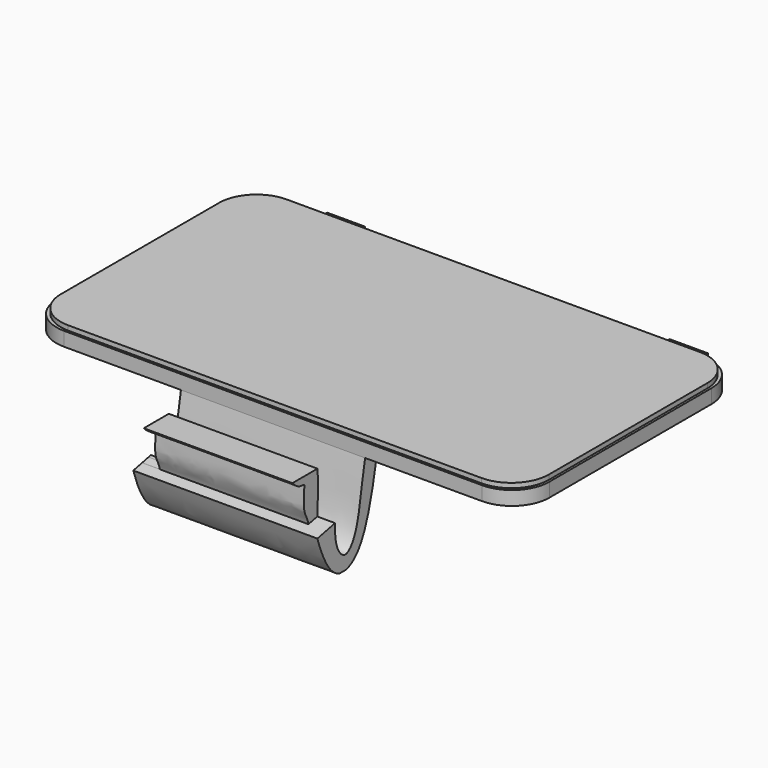
from build123d import *

# Parameters (mm, degrees)
F1_DEPTH  = 1.5
F3_DEPTH  = 0.5
F4_W      = 4.08
F4_H      = 3
F4_H_2    = 2
F5_DEPTH  = 2.15
F4_W_2    = 19.71
F4_H_3    = 8.35
F4_H_4    = 1.65
F6_DEPTH  = 9.5
F8_DEPTH  = 25.4
F9_DEPTH  = 25.4
F10_DEPTH = 25.4
F11_DEPTH = 25.4
F12_DEPTH = 1.9
F14_DEPTH = 1.9
F15_R     = 0.5


with BuildPart() as f1:
    # F0 (on Top) → F1 (new body)
    with BuildSketch(Plane.XY):
        with BuildLine():
            ThreePointArc((26.375, 10.85), (25.2034271247, 13.6784271247), (22.375, 14.85))
            Line((22.375, 14.85), (-22.375, 14.85))
            ThreePointArc((-22.375, 14.85), (-25.2034271247, 13.6784271247), (-26.375, 10.85))
            Line((-26.375, 10.85), (-26.375, -10.85))
            ThreePointArc((-26.375, -10.85), (-25.2034271247, -13.6784271247), (-22.375, -14.85))
            Line((-22.375, -14.85), (22.375, -14.85))
            ThreePointArc((22.375, -14.85), (25.2034271247, -13.6784271247), (26.375, -10.85))
            Line((26.375, -10.85), (26.375, 10.85))
        make_face()
    extrude(amount=F1_DEPTH)

    # F2 (on face) → F3 (join)
    with BuildSketch(Plane.XY.offset(1.5)):
        with BuildLine():
            ThreePointArc((26.125, 10.6), (24.9534271247, 13.4284271247), (22.125, 14.6))
            Line((22.125, 14.6), (-22.125, 14.6))
            ThreePointArc((-22.125, 14.6), (-24.9534271247, 13.4284271247), (-26.125, 10.6))
            Line((-26.125, 10.6), (-26.125, -10.6))
            ThreePointArc((-26.125, -10.6), (-24.9534271247, -13.4284271247), (-22.125, -14.6))
            Line((-22.125, -14.6), (22.125, -14.6))
            ThreePointArc((22.125, -14.6), (24.9534271247, -13.4284271247), (26.125, -10.6))
            Line((26.125, -10.6), (26.125, 10.6))
        make_face()
    extrude(amount=F3_DEPTH)

    # F4 (on face) → F5 (join)
    with BuildSketch(Plane.XY):
        with Locations((-18.335, 16.35)):
            Rectangle(F4_W, F4_H)
        with Locations((-18.335, 13.85)):
            Rectangle(F4_W, F4_H_2)
        with Locations((18.335, 13.85)):
            Rectangle(F4_W, F4_H_2)
        with Locations((18.335, 16.35)):
            Rectangle(F4_W, F4_H)
    extrude(amount=-F5_DEPTH)

    # F4 (on face) → F6 (join)
    with BuildSketch(Plane.XY):
        with Locations((0, -19.025)):
            Rectangle(F4_W_2, F4_H_3)
        with Locations((0, -14.025)):
            Rectangle(F4_W_2, F4_H_4)
    extrude(amount=-F6_DEPTH)

    # F7 (on face) → F8 (cut)
    with BuildSketch(Plane.YZ.offset(9.855)):
        with BuildLine():
            add(Edge.make_bspline(
                [(-18.2, -9.5), (-19.0467439554, -9.3105263347), (-20.1329314913, -7.9995740948), (-20.9745336298, -5.8262032925), (-21.2309185806, -5)],
                knots=[0.5048432027, 0.5048432027, 0.5048432027, 0.5048432027, 0.6991234522, 0.8042040894, 0.8042040894, 0.8042040894, 0.8042040894], degree=3))
            add(Edge.make_bspline(
                [(-21.2309185806, -5), (-21.7086386079, -3.4605420158), (-22.0508473288, -1.7012665692), (-22.2, 0)],
                knots=[0.8042040894, 0.8042040894, 0.8042040894, 0.8042040894, 1, 1, 1, 1], degree=3))
            Line((-22.2, 0), (-23.2, 0))
            Line((-23.2, 0), (-23.2, -9.5))
            Line((-23.2, -9.5), (-18.2, -9.5))
        make_face()
    extrude(amount=-F8_DEPTH, mode=Mode.SUBTRACT)

    # F7 (on face) → F9 (cut)
    with BuildSketch(Plane.YZ.offset(9.855)):
        with BuildLine():
            Line((-14.85, 0), (-18.85, 0))
            add(Edge.make_bspline(
                [(-18.8713932454, -4.5), (-18.8407563671, -3.1458271018), (-18.6661081701, -1.5784759436), (-18.85, 0)],
                knots=[0.789016397, 0.789016397, 0.789016397, 0.789016397, 1, 1, 1, 1], degree=3))
            add(Edge.make_bspline(
                [(-14.85, 0), (-15.4145938047, -2.6608863681), (-15.6218993367, -6.3008263141), (-17.5538748145, -8.6715731519), (-18.8298088893, -6.876353813), (-18.8868431725, -5.1828983108), (-18.8713932454, -4.5)],
                knots=[0, 0, 0, 0, 0.3263667999, 0.5024195639, 0.6826190926, 0.789016397, 0.789016397, 0.789016397, 0.789016397], degree=3))
        make_face()
    extrude(amount=-F9_DEPTH, mode=Mode.SUBTRACT)

    # F7 (on face) → F10 (cut)
    with BuildSketch(Plane.YZ.offset(9.855)):
        with BuildLine():
            add(Edge.make_bspline(
                [(-13.2, 0), (-13.822723688, -3.2937158649), (-14.7625971483, -7.9965886058), (-16.8744215828, -9.380788847), (-17.4416645725, -9.5)],
                knots=[0, 0, 0, 0, 0.3258242382, 0.4488307078, 0.4488307078, 0.4488307078, 0.4488307078], degree=3))
            Line((-17.4416645725, -9.5), (-13.2, -9.5))
            Line((-13.2, -9.5), (-13.2, 0))
        make_face()
    extrude(amount=-F10_DEPTH, mode=Mode.SUBTRACT)

    # F7 (on face) → F11 (cut)
    with BuildSketch(Plane.YZ.offset(9.855)):
        with BuildLine():
            add(Edge.make_bspline(
                [(-21.2309185806, -5), (-21.7086386079, -3.4605420158), (-22.0508473288, -1.7012665692), (-22.2, 0)],
                knots=[0.8042040894, 0.8042040894, 0.8042040894, 0.8042040894, 1, 1, 1, 1], degree=3))
            Line((-21.2309185806, -5), (-20.051155913, -4.75))
            add(Edge.make_bspline(
                [(-20.6, -0.8051507757), (-20.6309029539, -1.5331994881), (-20.8508854026, -3.4899190921), (-20.1828452771, -4.0737474943), (-20.051155913, -4.75)],
                knots=[0, 0, 0, 0, 0.5578277519, 1, 1, 1, 1], degree=3))
            add(Edge.make_bspline(
                [(-22.2, 0), (-22.021752265, -0.1914355168), (-21.34457939, -0.8364756071), (-20.8800740764, -0.7184244385), (-20.6, -0.8051507757)],
                knots=[0, 0, 0, 0, 0.5439991963, 1, 1, 1, 1], degree=3))
        make_face()
    extrude(amount=-F11_DEPTH, mode=Mode.SUBTRACT)

    # F7 (on face) → F12 (cut)
    with BuildSketch(Plane.YZ.offset(9.855)):
        with BuildLine():
            Line((-18.85, 0), (-22.2, 0))
            add(Edge.make_bspline(
                [(-22.2, 0), (-22.021752265, -0.1914355168), (-21.34457939, -0.8364756071), (-20.8800740764, -0.7184244385), (-20.6, -0.8051507757)],
                knots=[0, 0, 0, 0, 0.5439991963, 1, 1, 1, 1], degree=3))
            add(Edge.make_bspline(
                [(-20.6, -0.8051507757), (-20.6309029539, -1.5331994881), (-20.8508854026, -3.4899190921), (-20.1828452771, -4.0737474943), (-20.051155913, -4.75)],
                knots=[0, 0, 0, 0, 0.5578277519, 1, 1, 1, 1], degree=3))
            Line((-20.051155913, -4.75), (-18.8713932454, -4.5))
            add(Edge.make_bspline(
                [(-18.8713932454, -4.5), (-18.8407563671, -3.1458271018), (-18.6661081701, -1.5784759436), (-18.85, 0)],
                knots=[0.789016397, 0.789016397, 0.789016397, 0.789016397, 1, 1, 1, 1], degree=3))
        make_face()
    extrude(amount=-F12_DEPTH, mode=Mode.SUBTRACT)

    # F13 (on face) → F14 (cut)
    with BuildSketch(Plane(origin=(-9.855, 0, 0), x_dir=(0, -1, 0), z_dir=(-1, 0, 0))):
        with BuildLine():
            Line((20.0378884491, -4.7471885312), (20.051155913, -4.75))
            add(Edge.make_bspline(
                [(20.051155913, -4.75), (20.0589857611, -4.7097920877), (20.0674564332, -4.6697547253), (20.0765868052, -4.629908391), (20.0863933528, -4.5902740901), (20.0968875724, -4.5508725034), (20.1080734026, -4.5117231353), (20.1418817725, -4.4009968751), (20.1661686112, -4.3300403811), (20.1927551228, -4.2601282228), (20.2214794477, -4.1913122549), (20.2520262571, -4.1235210989), (20.2838500374, -4.0565219368), (20.3232108532, -3.9757663577), (20.3301650097, -3.9615765963), (20.3371409196, -3.9474033553), (20.3441319527, -3.9332429305), (20.3511312875, -3.9190914551), (20.3581319113, -3.9049448998), (20.3651266201, -3.8907990727)],
                knots=[0, 0, 0, 0, 0, 0, 0, 0, 0.0701472659, 0.0701472659, 0.0701472659, 0.0701472659, 0.0701472659, 0.0701472659, 0.1997739124, 0.1997739124, 0.1997739124, 0.1997739124, 0.1997739124, 0.1997739124, 0.227453691, 0.227453691, 0.227453691, 0.227453691, 0.227453691, 0.227453691, 0.227453691, 0.227453691], degree=7))
            add(Edge.make_bspline(
                [(20.3651266201, -3.8907990727), (20.2923732044, -3.9469893956), (20.0498312814, -4.1600578166), (19.9785290709, -4.465871509), (20.0378884491, -4.7471885312)],
                knots=[3.3352473479, 3.3352473479, 3.3352473479, 3.3352473479, 3.6014620339, 4.288683164, 4.288683164, 4.288683164, 4.288683164], degree=3))
        make_face()
        with BuildLine():
            Line((19.1865132018, -4.5667761333), (20.0378884491, -4.7471885312))
            add(Edge.make_bspline(
                [(20.3651266201, -3.8907990727), (20.2923732044, -3.9469893956), (20.0498312814, -4.1600578166), (19.9785290709, -4.465871509), (20.0378884491, -4.7471885312)],
                knots=[3.3352473479, 3.3352473479, 3.3352473479, 3.3352473479, 3.6014620339, 4.288683164, 4.288683164, 4.288683164, 4.288683164], degree=3))
            add(Edge.make_bspline(
                [(20.3651266201, -3.8907990727), (20.3652925358, -3.8904635312), (20.3654584482, -3.8901279902), (20.3656243571, -3.8897924495), (20.3657902625, -3.889456909), (20.3659561644, -3.8891213689), (20.3661220625, -3.8887858289), (20.3713416007, -3.8782287262), (20.3763917236, -3.8680073132), (20.3814356082, -3.8577844748), (20.3864705184, -3.8475586358), (20.3914936992, -3.8373282211), (20.3965023768, -3.8270916558), (20.4144692424, -3.7902165332), (20.4273277463, -3.7635338368), (20.4400206781, -3.7367712884), (20.4524989775, -3.709902642), (20.4647148079, -3.6829043352), (20.4766232471, -3.655756431), (20.5067795166, -3.5845105727), (20.5244774515, -3.5401460021), (20.541104477, -3.4952960694), (20.5565213512, -3.4499316007), (20.5706349892, -3.4040539743), (20.5833986563, -3.3576957084), (20.5998748454, -3.2900950162), (20.6046813043, -3.2691903931), (20.609204773, -3.2482009599), (20.6134948517, -3.227146708), (20.6175398341, -3.2060269198), (20.6213657385, -3.1848526801), (20.6372039955, -3.091846631), (20.6470136755, -3.0195059493), (20.6548666939, -2.9467874693), (20.6610708494, -2.8738168031), (20.6658588693, -2.8006775838), (20.6694244023, -2.7274178583), (20.6755601658, -2.5469844123), (20.6769210939, -2.4397334438), (20.6764794737, -2.3323859939), (20.6745662387, -2.2250049078), (20.6714409356, -2.1176310351), (20.6673316749, -2.0102860121), (20.660478022, -1.8599303262), (20.6583902963, -1.8168947561), (20.6561900649, -1.7738671435), (20.6538900562, -1.7308485214), (20.6515027419, -1.6878398889), (20.649040571, -1.6448422291), (20.6465162034, -1.6018565276)],
                knots=[0.227453691, 0.227453691, 0.227453691, 0.227453691, 0.227453691, 0.227453691, 0.227453691, 0.227453691, 0.2281102601, 0.2281102601, 0.2281102601, 0.2281102601, 0.2281102601, 0.2281102601, 0.24811135, 0.24811135, 0.24811135, 0.24811135, 0.24811135, 0.24811135, 0.3001057386, 0.3001057386, 0.3001057386, 0.3001057386, 0.3001057386, 0.3001057386, 0.3837391607, 0.3837391607, 0.3837391607, 0.3837391607, 0.3837391607, 0.3837391607, 0.4209624028, 0.4209624028, 0.4209624028, 0.4209624028, 0.4209624028, 0.4209624028, 0.5468509231, 0.5468509231, 0.5468509231, 0.5468509231, 0.5468509231, 0.5468509231, 0.7305556094, 0.7305556094, 0.7305556094, 0.7305556094, 0.7305556094, 0.7305556094, 0.8042380207, 0.8042380207, 0.8042380207, 0.8042380207, 0.8042380207, 0.8042380207, 0.8042380207, 0.8042380207], degree=7))
            add(Edge.make_bspline(
                [(20.6, -0.8051507757), (20.5613649055, -1.0322758666), (20.5772163889, -1.2973036751), (20.6410101063, -1.5787167701), (20.6465162034, -1.6018565276)],
                knots=[0, 0, 0, 0, 0.7282402744, 0.7931964139, 0.7931964139, 0.7931964139, 0.7931964139], degree=3))
            add(Edge.make_bspline(
                [(20.9991057889, -0.7416468993), (20.9592728425, -0.7301565498), (20.8220313096, -0.699983524), (20.6903609526, -0.7384588517), (20.6, -0.8051507757)],
                knots=[1.5561655905, 1.5561655905, 1.5561655905, 1.5561655905, 1.6760652117, 1.9692595941, 1.9692595941, 1.9692595941, 1.9692595941], degree=3))
            add(Edge.make_bspline(
                [(20.9991057889, -0.7416468993), (21.0018159449, -0.7414031777), (21.0045257326, -0.7411578671), (21.0072351577, -0.740910824), (21.0099442255, -0.7406619047), (21.0126529413, -0.7404109655), (21.0153613103, -0.7401578625), (21.0180693376, -0.7399024515), (21.0375384991, -0.7380483329), (21.0542867078, -0.7363581789), (21.0710231722, -0.7345401107), (21.0877483889, -0.7325603549), (21.104461824, -0.7303860252), (21.1211619051, -0.7279857666), (21.137846013, -0.7253304002), (21.1787532558, -0.7181211815), (21.2029571594, -0.7132526524), (21.22710557, -0.7077075247), (21.251178971, -0.7014182819), (21.2751551853, -0.6943343572), (21.2990094679, -0.6864244774), (21.3227144456, -0.6776773383), (21.3912145071, -0.6497923866), (21.43549452, -0.628448223), (21.4790992276, -0.6048089523), (21.5220195614, -0.5793468432), (21.5642587373, -0.5524077139), (21.6058418345, -0.5242508404), (21.6468131809, -0.4950496177), (21.7124884675, -0.4460965112), (21.737506514, -0.4269266559), (21.7622997408, -0.4074426066), (21.7868715943, -0.3876760423), (21.8112238209, -0.36765495), (21.835356514, -0.3474044919), (21.8592681613, -0.3269478723), (21.9071685483, -0.285208783), (21.9311359694, -0.2639277816), (21.9548620733, -0.2424817194), (21.9783439347, -0.2208903242), (22.0015734403, -0.1991751296), (22.0245346788, -0.1773623394), (22.0472039759, -0.1554833002), (22.0695454706, -0.1335784594)],
                knots=[0.2229980472, 0.2229980472, 0.2229980472, 0.2229980472, 0.2229980472, 0.2229980472, 0.2229980472, 0.2229980472, 0.2229980472, 0.235216929, 0.235216929, 0.235216929, 0.235216929, 0.235216929, 0.235216929, 0.235216929, 0.310855725, 0.310855725, 0.310855725, 0.310855725, 0.310855725, 0.310855725, 0.310855725, 0.4208919894, 0.4208919894, 0.4208919894, 0.4208919894, 0.4208919894, 0.4208919894, 0.4208919894, 0.6312529006, 0.6312529006, 0.6312529006, 0.6312529006, 0.6312529006, 0.6312529006, 0.6312529006, 0.7626298331, 0.7626298331, 0.7626298331, 0.7626298331, 0.7626298331, 0.7626298331, 0.7626298331, 0.8969203539, 0.8969203539, 0.8969203539, 0.8969203539, 0.8969203539, 0.8969203539, 0.8969203539, 0.8969203539, 0.8969203539], degree=8))
            add(Edge.make_bspline(
                [(22.2, 0), (22.1557451499, -0.0395755652), (22.1122969775, -0.0840429257), (22.0695454706, -0.1335784594)],
                knots=[0, 0, 0, 0, 0.1902494763, 0.1902494763, 0.1902494763, 0.1902494763], degree=3))
            Line((22.2, 0), (18.85, 0))
            add(Edge.make_bspline(
                [(18.85, 0), (18.8041285234, -0.3937479028), (18.7758085808, -0.7894835109), (18.7623451707, -1.1860157865), (18.7608009494, -1.5825878818), (18.7682857506, -1.9788864083), (18.785468482, -2.4902466637), (18.7898321752, -2.6054346786), (18.7946093212, -2.7206051301), (18.799718478, -2.8357595323), (18.8050745896, -2.9509007431), (18.8123523874, -3.1028850541), (18.8141331269, -3.1397361515), (18.8159270051, -3.1765864439), (18.8177310212, -3.2134360696), (18.8195421073, -3.2502851717), (18.8213571287, -3.2871338975)],
                knots=[0, 0, 0, 0, 0, 0, 0, 0.5278695798, 0.5278695798, 0.5278695798, 0.5278695798, 0.5278695798, 0.6813794986, 0.6813794986, 0.6813794986, 0.6813794986, 0.6813794986, 0.7305156181, 0.7305156181, 0.7305156181, 0.7305156181, 0.7305156181, 0.7305156181, 0.7305156181], degree=6))
            add(Edge.make_bspline(
                [(19.1865132018, -4.5667761333), (19.0849025154, -4.1217046012), (18.9454363675, -3.7042708733), (18.8213571287, -3.2871338975)],
                knots=[15.3483435034, 15.3483435034, 15.3483435034, 15.3483435034, 16.7073787198, 16.7073787198, 16.7073787198, 16.7073787198], degree=3))
        make_face()
        with BuildLine():
            Line((18.8713932454, -4.5), (19.1865132018, -4.5667761333))
            add(Edge.make_bspline(
                [(19.1865132018, -4.5667761333), (19.0849025154, -4.1217046012), (18.9454363675, -3.7042708733), (18.8213571287, -3.2871338975)],
                knots=[15.3483435034, 15.3483435034, 15.3483435034, 15.3483435034, 16.7073787198, 16.7073787198, 16.7073787198, 16.7073787198], degree=3))
            add(Edge.make_bspline(
                [(18.8213571287, -3.2871338975), (18.8234567809, -3.3297612222), (18.8255616994, -3.3723880433), (18.8276670315, -3.4150145889), (18.8297678045, -3.4576410948), (18.8318589258, -3.5002678049), (18.8369559593, -3.6049138465), (18.8399452005, -3.6669336481), (18.8428868298, -3.7289551465), (18.8457639747, -3.7909790554), (18.8485589666, -3.8530060314), (18.8554869159, -4.0125032039), (18.8594720136, -4.1099784592), (18.8631366493, -4.2074652335), (18.8664032639, -4.3049647894), (18.8691868781, -4.4024769185), (18.8713932454, -4.5)],
                knots=[0.7305156181, 0.7305156181, 0.7305156181, 0.7305156181, 0.7305156181, 0.7305156181, 0.7305156181, 0.7873572394, 0.7873572394, 0.7873572394, 0.7873572394, 0.7873572394, 0.8700569312, 0.8700569312, 0.8700569312, 0.8700569312, 0.8700569312, 1, 1, 1, 1, 1, 1, 1], degree=6))
        make_face()
        with BuildLine():
            add(Edge.make_bspline(
                [(20.6, -0.8051507757), (20.5613649055, -1.0322758666), (20.5772163889, -1.2973036751), (20.6410101063, -1.5787167701), (20.6465162034, -1.6018565276)],
                knots=[0, 0, 0, 0, 0.7282402744, 0.7931964139, 0.7931964139, 0.7931964139, 0.7931964139], degree=3))
            add(Edge.make_bspline(
                [(20.6465162034, -1.6018565276), (20.6454874073, -1.5843378735), (20.6444482807, -1.5668212056), (20.6433996806, -1.5493065906), (20.6423424697, -1.5317940952), (20.6412775194, -1.5142837865), (20.6402057118, -1.496775732), (20.6346132485, -1.4059397594), (20.6299941701, -1.3326518291), (20.6253361607, -1.2594097858), (20.6207110068, -1.1862201726), (20.6161978814, -1.1130924918), (20.6118930639, -1.0400403627), (20.6066693408, -0.9439168342), (20.6054447252, -0.9207596352), (20.6042585866, -0.8976129266), (20.6031155769, -0.8744775635), (20.6020208919, -0.8513545797), (20.6009802717, -0.8282451869), (20.6, -0.8051507757)],
                knots=[0.8042380207, 0.8042380207, 0.8042380207, 0.8042380207, 0.8042380207, 0.8042380207, 0.8042380207, 0.8042380207, 0.8342669986, 0.8342669986, 0.8342669986, 0.8342669986, 0.8342669986, 0.8342669986, 0.9600562049, 0.9600562049, 0.9600562049, 0.9600562049, 0.9600562049, 0.9600562049, 1, 1, 1, 1, 1, 1, 1, 1], degree=7))
        make_face()
        with BuildLine():
            add(Edge.make_bspline(
                [(20.9991057889, -0.7416468993), (20.9592728425, -0.7301565498), (20.8220313096, -0.699983524), (20.6903609526, -0.7384588517), (20.6, -0.8051507757)],
                knots=[1.5561655905, 1.5561655905, 1.5561655905, 1.5561655905, 1.6760652117, 1.9692595941, 1.9692595941, 1.9692595941, 1.9692595941], degree=3))
            add(Edge.make_bspline(
                [(20.6, -0.8051507757), (20.6357983312, -0.7940656436), (20.6717568885, -0.7844174379), (20.7077937642, -0.7761910472), (20.7438427247, -0.7693108375), (20.7798531645, -0.7636357507), (20.8157901974, -0.7589622849), (20.8516348851, -0.7550353533), (20.8965863081, -0.7506743043), (20.9057821139, -0.7498119471), (20.9149720884, -0.748974999), (20.9241563382, -0.7481584013), (20.93333501, -0.7473569911), (20.9425082907, -0.7465655013), (20.9516764072, -0.7457785607), (20.9656273652, -0.7445790375), (20.9704137565, -0.7441671385), (20.9751988374, -0.7437542175), (20.9799826436, -0.7433394936), (20.9847652094, -0.7429221844), (20.9895465679, -0.7425015061), (20.9943267509, -0.7420766732), (20.9991057889, -0.7416468993)],
                knots=[0, 0, 0, 0, 0, 0, 0, 0, 0, 0.1602137189, 0.1602137189, 0.1602137189, 0.1602137189, 0.1602137189, 0.1602137189, 0.1602137189, 0.2014515012, 0.2014515012, 0.2014515012, 0.2014515012, 0.2014515012, 0.2014515012, 0.2014515012, 0.2229980472, 0.2229980472, 0.2229980472, 0.2229980472, 0.2229980472, 0.2229980472, 0.2229980472, 0.2229980472, 0.2229980472], degree=8))
        make_face()
        with BuildLine():
            add(Edge.make_bspline(
                [(22.0695454706, -0.1335784594), (22.0819512565, -0.1214151387), (22.0942559691, -0.1092438625), (22.1064534685, -0.0970715557), (22.1185364564, -0.0849060086), (22.130496242, -0.0727560855), (22.1423223785, -0.0606320358), (22.1540020519, -0.0485460024), (22.1699223859, -0.0319121785), (22.1743015208, -0.0273196696), (22.1786553865, -0.0227363366), (22.1829828315, -0.0181632572), (22.1872825506, -0.013601651), (22.1915530853, -0.0090528797), (22.1957928235, -0.0045184474), (22.2, 0)],
                knots=[0.8969203539, 0.8969203539, 0.8969203539, 0.8969203539, 0.8969203539, 0.8969203539, 0.8969203539, 0.8969203539, 0.8969203539, 0.9714891983, 0.9714891983, 0.9714891983, 0.9714891983, 0.9714891983, 0.9714891983, 0.9714891983, 1, 1, 1, 1, 1, 1, 1, 1, 1], degree=8))
            add(Edge.make_bspline(
                [(22.2, 0), (22.1557451499, -0.0395755652), (22.1122969775, -0.0840429257), (22.0695454706, -0.1335784594)],
                knots=[0, 0, 0, 0, 0.1902494763, 0.1902494763, 0.1902494763, 0.1902494763], degree=3))
        make_face()
    extrude(amount=-F14_DEPTH, mode=Mode.SUBTRACT)

    # F15
    f15_edges = [f1.edges().sort_by_distance(p)[0] for p in [
        (18.335, 17.85, -2.15),
        (-18.335, 17.85, -2.15),
    ]]
    fillet(f15_edges, radius=F15_R)


solid = f1.part
